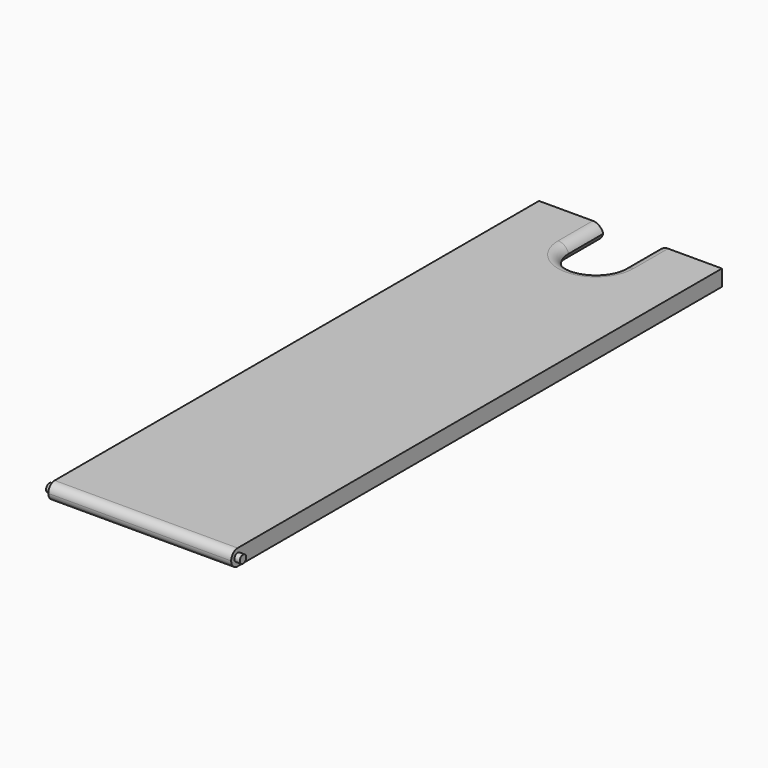
from build123d import *

# Parameters (mm, degrees)
F0_W          = 43.18
F0_H          = 144.78
F1_DEPTH      = 3.81
F3_DEPTH      = 25.4
F4_T3_DEPTH   = 16.5585234346
F4_T6_DEPTH   = 16.5585234346
F4_T9_ANGLE   = 180
F4_T12_DEPTH  = 16.5585234346
F4_T15_ANGLE  = 180
F4_T18_DEPTH  = 16.5585234346
F5_R          = 1.90499
F6_R          = 0.9525
F7_DEPTH      = 1.27
F7_DEPTH_BACK = 44.45


# Not quite as in the source:
# - a fillet or chamfer that OpenCascade refuses, or shapes differently, is made with other operations: its cross-section is extruded or revolved along the edge and cut away or added
# - a fillet or chamfer is up to 0.001 mm smaller than in the source, because OpenCascade refuses the exact size


with BuildPart() as f1:
    # F0 (on Top) → F1 (new body)
    with BuildSketch(Plane.XY):
        with Locations((-6.204857491, -4.3873040367)):
            Rectangle(F0_W, F0_H)
    extrude(amount=F1_DEPTH)

    # F2 (on face) → F3 (cut)
    with BuildSketch(Plane.XY.offset(3.81)):
        with BuildLine():
            ThreePointArc((0.145142509, 57.7941725286), (-6.204857491, 64.1441725286), (-12.554857491, 57.7941725286))
            Line((-12.554857491, 57.7941725286), (0.145142509, 57.7941725286))
        make_face()
        with BuildLine():
            Line((0.145142509, 68.0026959633), (-12.554857491, 68.0026959633))
            Line((-12.554857491, 68.0026959633), (-12.554857491, 57.7941725286))
            ThreePointArc((-12.554857491, 57.7941725286), (-6.204857491, 64.1441725286), (0.145142509, 57.7941725286))
            Line((0.145142509, 57.7941725286), (0.145142509, 68.0026959633))
        make_face()
        with BuildLine():
            Line((0.145142509, 57.7941725286), (-12.554857491, 57.7941725286))
            ThreePointArc((-12.554857491, 57.7941725286), (-6.204857491, 51.4441725286), (0.145142509, 57.7941725286))
        make_face()
    extrude(amount=-F3_DEPTH, mode=Mode.SUBTRACT)

    # F4: fillet of radius 2.54 on 2 edges, made by hand


with BuildPart() as f4_tool1:
    # F4_s2 → F4_t3 (new body)
    with BuildSketch(Plane.XZ.offset(-74.3526959633)):
        with BuildLine():
            ThreePointArc((-15.094857491, 3.81), (-13.2988062667, 3.0660512242), (-12.554857491, 1.27))
            Line((-12.554857491, 1.27), (-12.554857491, 3.81))
            Line((-12.554857491, 3.81), (-15.094857491, 3.81))
        make_face()
    extrude(amount=F4_T3_DEPTH)


with BuildPart() as f4_tool4:
    # F4_s5 → F4_t6 (new body)
    with BuildSketch(Plane.XZ.offset(-74.3526959633)):
        with BuildLine():
            ThreePointArc((-15.094857491, 0), (-13.2988062667, 0.7439487758), (-12.554857491, 2.54))
            Line((-12.554857491, 2.54), (-12.554857491, 0))
            Line((-12.554857491, 0), (-15.094857491, 0))
        make_face()
    extrude(amount=F4_T6_DEPTH)


with BuildPart() as f4_tool7:
    # F4_s8 → F4_t9 (revolve)
    with BuildSketch(Plane.XZ.offset(-57.7941725286)):
        with BuildLine():
            ThreePointArc((-15.094857491, 0), (-13.2988062667, 0.7439487758), (-12.554857491, 2.54))
            Line((-12.554857491, 2.54), (-12.554857491, 0))
            Line((-12.554857491, 0), (-15.094857491, 0))
        make_face()
    revolve(axis=Axis((-6.204857491, 57.7941725286, 0), (0, 0, 1)), revolution_arc=F4_T9_ANGLE)


with BuildPart() as f4_tool10:
    # F4_s11 → F4_t12 (new body)
    with BuildSketch(Plane.XZ.offset(-57.7941725286)):
        with BuildLine():
            ThreePointArc((2.685142509, 0), (0.8890912848, 0.7439487758), (0.145142509, 2.54))
            Line((0.145142509, 2.54), (0.145142509, 0))
            Line((0.145142509, 0), (2.685142509, 0))
        make_face()
    extrude(amount=-F4_T12_DEPTH)


with BuildPart() as f4_tool13:
    # F4_s14 → F4_t15 (revolve)
    with BuildSketch(Plane.XZ.offset(-57.7941725286)):
        with BuildLine():
            ThreePointArc((-15.094857491, 3.81), (-13.2988062667, 3.0660512242), (-12.554857491, 1.27))
            Line((-12.554857491, 1.27), (-12.554857491, 3.81))
            Line((-12.554857491, 3.81), (-15.094857491, 3.81))
        make_face()
    revolve(axis=Axis((-6.204857491, 57.7941725286, 3.81), (0, 0, 1)), revolution_arc=F4_T15_ANGLE)


with BuildPart() as f4_tool16:
    # F4_s17 → F4_t18 (new body)
    with BuildSketch(Plane.XZ.offset(-57.7941725286)):
        with BuildLine():
            ThreePointArc((2.685142509, 3.81), (0.8890912848, 3.0660512242), (0.145142509, 1.27))
            Line((0.145142509, 1.27), (0.145142509, 3.81))
            Line((0.145142509, 3.81), (2.685142509, 3.81))
        make_face()
    extrude(amount=-F4_T18_DEPTH)


with BuildPart() as f1_1:
    add(f1.part)

    # F4_t19: cut F4_tool1, F4_tool4, F4_tool7, F4_tool10, F4_tool13, F4_tool16
    add([f4_tool1.part, f4_tool4.part, f4_tool7.part, f4_tool10.part, f4_tool13.part, f4_tool16.part], mode=Mode.SUBTRACT)

    # F5 (radius 1.905 in the source; OpenCascade refuses exactly that, so slightly less here)
    f5_edges = [f1_1.edges().sort_by_distance(p)[0] for p in [
        (-6.204857, -76.777304, 3.81),
        (-6.204857, -76.777304, 0),
    ]]
    fillet(f5_edges, radius=F5_R)

    # F6 (on face) → F7 (join, two sides)
    with BuildSketch(Plane(origin=(-27.794857491, 0, 0), x_dir=(0, -1, 0), z_dir=(-1, 0, 0))) as f7_sk:
        with Locations((74.8723040367, 1.905)):
            Circle(F6_R)
    extrude(amount=F7_DEPTH)
    extrude(f7_sk.sketch, amount=-F7_DEPTH_BACK)


solid = f1_1.part
